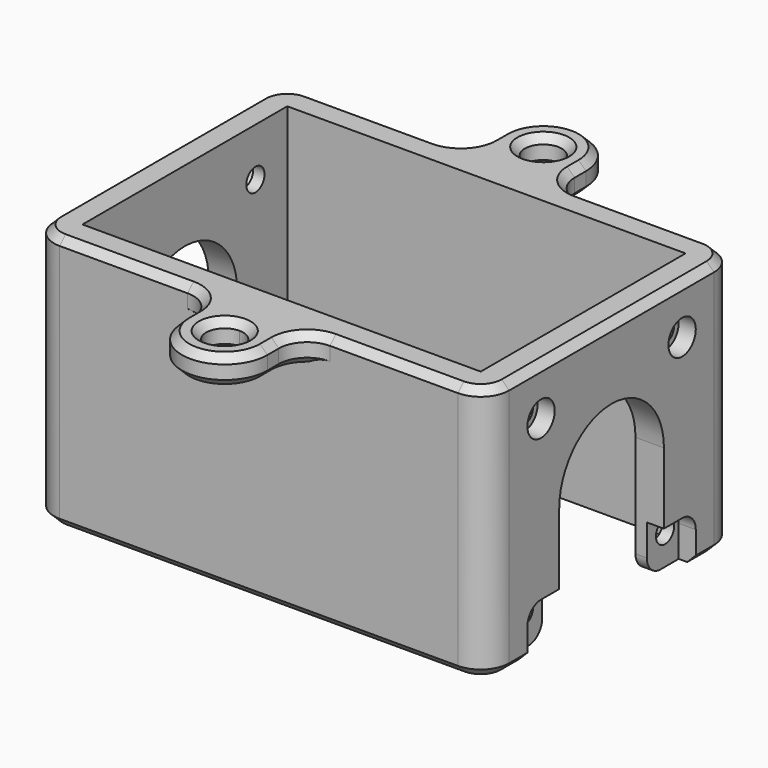
from build123d import *

# Parameters (mm, degrees)
F0_W          = 70
F0_H          = 45
F1_DEPTH      = 45
F2_R          = 2
F3_DEPTH      = 40.001
F3_DEPTH_BACK = 40.001
F5_R          = 3
F6_DEPTH      = 3
F7_R          = 3
F8_DEPTH      = 3
F9_R          = 3
F10_SIZE      = 1.5
F12_DEPTH     = 5
F13_R         = 5
F14_T1_DEPTH  = 22.5
F14_T3_DEPTH  = 22.5
F14_T5_DEPTH  = 2.5
F14_T7_DEPTH  = 45
F14_T9_DEPTH  = 2.5
F14_T16_ANGLE = 180
F14_T22_ANGLE = 128.3255006626
F14_T27_ANGLE = 90
F14_T29_ANGLE = 90
F14_T31_ANGLE = 180
F14_T33_ANGLE = 90
F14_T35_ANGLE = 90
F14_T37_ANGLE = 90
F14_T39_ANGLE = 90
F14_T41_ANGLE = 180
F14_T43_ANGLE = 90
F14_T45_ANGLE = 90
F14_T49_ANGLE = 128.3255006626
F14_T52_ANGLE = 180
F14_T56_ANGLE = 128.3255006626
F14_T61_ANGLE = 128.3255006626


# Not quite as in the source:
# - a fillet or chamfer that OpenCascade refuses, or shapes differently, is made with other operations: its cross-section is extruded or revolved along the edge and cut away or added


with BuildPart() as f1:
    # F0 (on Top) → F1 (new body)
    with BuildSketch(Plane.XY):
        with BuildLine():
            ThreePointArc((40, 22.5), (38.5355339059, 26.0355339059), (35, 27.5))
            Line((35, 27.5), (-35, 27.5))
            ThreePointArc((-35, 27.5), (-38.5355339059, 26.0355339059), (-40, 22.5))
            Line((-40, 22.5), (-40, -22.5))
            ThreePointArc((-40, -22.5), (-38.5355339059, -26.0355339059), (-35, -27.5))
            Line((-35, -27.5), (35, -27.5))
            ThreePointArc((35, -27.5), (38.5355339059, -26.0355339059), (40, -22.5))
            Line((40, -22.5), (40, 22.5))
        make_face()
        Rectangle(F0_W, F0_H, mode=Mode.SUBTRACT)
    extrude(amount=F1_DEPTH)

    # F2 (on Right) → F3 (cut, two sides)
    with BuildSketch(Plane.YZ) as f3_sk:
        with Locations((15.5, 36.5)):
            Circle(F2_R)
        with Locations((-15.5, 36.5)):
            Circle(F2_R)
        with Locations((15.5, 5.5)):
            Circle(F2_R)
        with Locations((-15.5, 5.5)):
            Circle(F2_R)
        with BuildLine():
            Line((11.5, 0), (11.5, 21))
            ThreePointArc((11.5, 21), (0, 32.5), (-11.5, 21))
            Line((-11.5, 21), (-11.5, 0))
            Line((-11.5, 0), (11.5, 0))
        make_face()
    extrude(amount=-F3_DEPTH, mode=Mode.SUBTRACT)
    extrude(f3_sk.sketch, amount=F3_DEPTH_BACK, mode=Mode.SUBTRACT)

    # F5 (on face) → F6 (cut)
    with BuildSketch(Plane.YZ.offset(40)):
        with Locations((-15.5, 36.5)):
            Circle(F5_R)
        with Locations((15.5, 36.5)):
            Circle(F5_R)
        with BuildLine():
            ThreePointArc((-15.5, 8.5), (-17.6213203436, 7.6213203436), (-18.5, 5.5))
            Line((-18.5, 5.5), (-18.5, 0))
            Line((-18.5, 0), (-11.5, 0))
            Line((-11.5, 0), (-11.5, 8.5))
            Line((-11.5, 8.5), (-15.5, 8.5))
        make_face()
        with BuildLine():
            Line((15.5, 8.5), (11.5, 8.5))
            Line((11.5, 8.5), (11.5, 0))
            Line((11.5, 0), (18.5, 0))
            Line((18.5, 0), (18.5, 5.5))
            ThreePointArc((18.5, 5.5), (17.6213203436, 7.6213203436), (15.5, 8.5))
        make_face()
    extrude(amount=-F6_DEPTH, mode=Mode.SUBTRACT)

    # F7 (on face) → F8 (cut)
    with BuildSketch(Plane(origin=(-40, 0, 0), x_dir=(0, -1, 0), z_dir=(-1, 0, 0))):
        with Locations((-15.5, 36.5)):
            Circle(F7_R)
        with Locations((15.5, 36.5)):
            Circle(F7_R)
        with BuildLine():
            Line((11.5, 0), (18.5, 0))
            Line((18.5, 0), (18.5, 5.5))
            ThreePointArc((18.5, 5.5), (17.6213203436, 7.6213203436), (15.5, 8.5))
            Line((15.5, 8.5), (11.5, 8.5))
            Line((11.5, 8.5), (11.5, 0))
        make_face()
        with BuildLine():
            Line((-11.5, 8.5), (-15.5, 8.5))
            ThreePointArc((-15.5, 8.5), (-17.6213203436, 7.6213203436), (-18.5, 5.5))
            Line((-18.5, 5.5), (-18.5, 0))
            Line((-18.5, 0), (-11.5, 0))
            Line((-11.5, 0), (-11.5, 8.5))
        make_face()
    extrude(amount=-F8_DEPTH, mode=Mode.SUBTRACT)

    # F9
    f9_edges = [f1.edges().sort_by_distance(p)[0] for p in [
        (36, 11.5, 0),
        (-36, 11.5, 0),
        (-36, -11.5, 0),
        (36, -11.5, 0),
    ]]
    fillet(f9_edges, radius=F9_R)

    # F10
    f10_edges = [f1.edges().sort_by_distance(p)[0] for p in [
        (-40, 20.5, 0),
        (-38.535534, -26.035534, 0),
        (-40, -20.5, 0),
        (0, -27.5, 0),
        (38.535534, -26.035534, 0),
        (40, -20.5, 0),
        (40, 20.5, 0),
        (38.535534, 26.035534, 0),
        (0, 27.5, 0),
        (-38.535534, 26.035534, 0),
    ]]
    chamfer(f10_edges, length=F10_SIZE)

    # F11 (on face) → F12 (join)
    with BuildSketch(Plane.XY.offset(45)):
        with BuildLine():
            Line((-7.5, 27.5), (0, 27.5))
            Line((0, 27.5), (7.5, 27.5))
            Line((7.5, 27.5), (7.5, 35))
            ThreePointArc((7.5, 35), (0, 42.5), (-7.5, 35))
            Line((-7.5, 35), (-7.5, 27.5))
        make_face()
        with BuildLine():
            ThreePointArc((0, 31.75), (-2.2980970389, 37.2980970389), (3.25, 35))
            ThreePointArc((3.25, 35), (2.2980970389, 32.7019029611), (0, 31.75))
        make_face(mode=Mode.SUBTRACT)
        with BuildLine():
            Line((7.5, -22.5), (0, -22.5))
            Line((0, -22.5), (-7.5, -22.5))
            Line((-7.5, -22.5), (-7.5, -35))
            ThreePointArc((-7.5, -35), (0, -42.5), (7.5, -35))
            Line((7.5, -35), (7.5, -22.5))
        make_face()
        with BuildLine():
            ThreePointArc((3.25, -35), (-2.2980970389, -37.2980970389), (0, -31.75))
            ThreePointArc((0, -31.75), (2.2980970389, -32.7019029611), (3.25, -35))
        make_face(mode=Mode.SUBTRACT)
    extrude(amount=-F12_DEPTH)

    # F13
    f13_edges = [f1.edges().sort_by_distance(p)[0] for p in [
        (7.5, 27.5, 42.5),
        (-7.5, 27.5, 42.5),
        (-7.5, -27.5, 42.5),
        (7.5, -27.5, 42.5),
    ]]
    fillet(f13_edges, radius=F13_R)

    # F14: chamfer of 1.3 on 34 edges, made by hand

    # F14_s2 → F14_t1 (cut)
    with BuildSketch(Plane.YZ.offset(12.5)):
        Polygon((-27.5, 43.7), (-26.2, 45), (-27.5, 45), align=None)
        Polygon((26.2, 45), (27.5, 43.7), (27.5, 45), align=None)
    extrude(amount=F14_T1_DEPTH, mode=Mode.SUBTRACT)

    # F14_s4 → F14_t3 (cut)
    with BuildSketch(Plane.YZ.offset(-35)):
        Polygon((-27.5, 43.7), (-26.2, 45), (-27.5, 45), align=None)
        Polygon((26.2, 45), (27.5, 43.7), (27.5, 45), align=None)
    extrude(amount=F14_T3_DEPTH, mode=Mode.SUBTRACT)

    # F14_s6 → F14_t5 (cut)
    with BuildSketch(Plane.XZ.offset(32.5)):
        Polygon((6.2, 45), (7.5, 43.7), (7.5, 45), align=None)
        Polygon((-6.2, 45), (-7.5, 43.7), (-7.5, 45), align=None)
        Polygon((-6.2, 40), (-7.5, 41.3), (-7.5, 40), align=None)
        Polygon((6.2, 40), (7.5, 41.3), (7.5, 40), align=None)
    extrude(amount=F14_T5_DEPTH, mode=Mode.SUBTRACT)

    # F14_s8 → F14_t7 (cut)
    with BuildSketch(Plane.XZ.offset(-22.5)):
        Polygon((38.7, 45), (40, 43.7), (40, 45), align=None)
        Polygon((-38.7, 45), (-40, 43.7), (-40, 45), align=None)
    extrude(amount=F14_T7_DEPTH, mode=Mode.SUBTRACT)

    # F14_s10 → F14_t9 (cut)
    with BuildSketch(Plane.XZ.offset(-35)):
        Polygon((6.2, 45), (7.5, 43.7), (7.5, 45), align=None)
        Polygon((-6.2, 45), (-7.5, 43.7), (-7.5, 45), align=None)
        Polygon((7.5, 41.3), (6.2, 40), (7.5, 40), align=None)
        Polygon((-7.5, 41.3), (-6.2, 40), (-7.5, 40), align=None)
    extrude(amount=F14_T9_DEPTH, mode=Mode.SUBTRACT)

    # F14_s11 → F14_t12 (revolve, cut)
    with BuildSketch(Plane.XZ.offset(35)):
        Polygon((4.55, 45), (3.25, 43.7), (3.25, 45), align=None)
    revolve(axis=Axis((0, -35, 45), (0, 0, -1)), mode=Mode.SUBTRACT)

    # F14_s13 → F14_t14 (revolve, cut)
    with BuildSketch(Plane.XZ.offset(-35)):
        Polygon((4.55, 45), (3.25, 43.7), (3.25, 45), align=None)
    revolve(axis=Axis((0, 35, 45), (0, 0, -1)), mode=Mode.SUBTRACT)

    # F14_s15 → F14_t16 (revolve, cut)
    with BuildSketch(Plane.XZ.offset(-35)):
        Polygon((7.5, 41.3), (6.2, 40), (7.5, 40), align=None)
    revolve(axis=Axis((0, 35, 40), (0, 0, 1)), revolution_arc=F14_T16_ANGLE, mode=Mode.SUBTRACT)

    # F14_s17 → F14_t18 (revolve, cut)
    with BuildSketch(Plane.XZ.offset(-35)):
        Polygon((3.25, 41.3), (4.55, 40), (3.25, 40), align=None)
    revolve(axis=Axis((0, 35, 40), (0, 0, -1)), mode=Mode.SUBTRACT)


with BuildPart() as f14_tool20:
    # F14_s21 → F14_t22 (revolve)
    with BuildSketch(Plane(origin=(-23.5039658434, -18.5793051911, 0), x_dir=(0, 0, 1), z_dir=(-0.7845004474, -0.6201282512, 0))):
        Polygon((40, -11.4446614013), (41.3, -12.7446614013), (40, -12.7446614013), align=None)
    revolve(axis=Axis((-12.5, -32.5, 40), (0, 0, -1)), revolution_arc=F14_T22_ANGLE)

    split(bisect_by=Plane.XZ.offset(27.5), keep=Keep.TOP)


with BuildPart() as f1_1:
    add(f1.part)

    # F14_t19: cut F14_tool20
    add(f14_tool20.part, mode=Mode.SUBTRACT)

    # F14_s24 → F14_t25 (revolve, cut)
    with BuildSketch(Plane.XZ.offset(35)):
        Polygon((4.55, 40), (3.25, 41.3), (3.25, 40), align=None)
    revolve(axis=Axis((0, -35, 40), (0, 0, -1)), mode=Mode.SUBTRACT)

    # F14_s26 → F14_t27 (revolve, cut)
    with BuildSketch(Plane.YZ.offset(12.5)):
        Polygon((-26.2, 45), (-27.5, 43.7), (-27.5, 45), align=None)
    revolve(axis=Axis((12.5, -32.5, 45), (0, 0, 1)), revolution_arc=F14_T27_ANGLE, mode=Mode.SUBTRACT)

    # F14_s28 → F14_t29 (revolve, cut)
    with BuildSketch(Plane.YZ.offset(35)):
        Polygon((-26.2, 45), (-27.5, 43.7), (-27.5, 45), align=None)
    revolve(axis=Axis((35, -22.5, 45), (0, 0, 1)), revolution_arc=F14_T29_ANGLE, mode=Mode.SUBTRACT)

    # F14_s30 → F14_t31 (revolve, cut)
    with BuildSketch(Plane.XZ.offset(35)):
        Polygon((-6.2, 45), (-7.5, 43.7), (-7.5, 45), align=None)
    revolve(axis=Axis((0, -35, 45), (0, 0, 1)), revolution_arc=F14_T31_ANGLE, mode=Mode.SUBTRACT)

    # F14_s32 → F14_t33 (revolve, cut)
    with BuildSketch(Plane.XZ.offset(-22.5)):
        Polygon((38.7, 45), (40, 43.7), (40, 45), align=None)
    revolve(axis=Axis((35, 22.5, 45), (0, 0, 1)), revolution_arc=F14_T33_ANGLE, mode=Mode.SUBTRACT)

    # F14_s34 → F14_t35 (revolve, cut)
    with BuildSketch(Plane.YZ.offset(-12.5)):
        Polygon((-26.2, 45), (-27.5, 43.7), (-27.5, 45), align=None)
    revolve(axis=Axis((-12.5, -32.5, 45), (0, 0, -1)), revolution_arc=F14_T35_ANGLE, mode=Mode.SUBTRACT)

    # F14_s36 → F14_t37 (revolve, cut)
    with BuildSketch(Plane.YZ.offset(12.5)):
        Polygon((26.2, 45), (27.5, 43.7), (27.5, 45), align=None)
    revolve(axis=Axis((12.5, 32.5, 45), (0, 0, -1)), revolution_arc=F14_T37_ANGLE, mode=Mode.SUBTRACT)

    # F14_s38 → F14_t39 (revolve, cut)
    with BuildSketch(Plane.XZ.offset(22.5)):
        Polygon((-38.7, 45), (-40, 43.7), (-40, 45), align=None)
    revolve(axis=Axis((-35, -22.5, 45), (0, 0, 1)), revolution_arc=F14_T39_ANGLE, mode=Mode.SUBTRACT)

    # F14_s40 → F14_t41 (revolve, cut)
    with BuildSketch(Plane.XZ.offset(-35)):
        Polygon((6.2, 45), (7.5, 43.7), (7.5, 45), align=None)
    revolve(axis=Axis((0, 35, 45), (0, 0, 1)), revolution_arc=F14_T41_ANGLE, mode=Mode.SUBTRACT)

    # F14_s42 → F14_t43 (revolve, cut)
    with BuildSketch(Plane.YZ.offset(-35)):
        Polygon((26.2, 45), (27.5, 43.7), (27.5, 45), align=None)
    revolve(axis=Axis((-35, 22.5, 45), (0, 0, 1)), revolution_arc=F14_T43_ANGLE, mode=Mode.SUBTRACT)

    # F14_s44 → F14_t45 (revolve, cut)
    with BuildSketch(Plane.YZ.offset(-12.5)):
        Polygon((26.2, 45), (27.5, 43.7), (27.5, 45), align=None)
    revolve(axis=Axis((-12.5, 32.5, 45), (0, 0, 1)), revolution_arc=F14_T45_ANGLE, mode=Mode.SUBTRACT)


with BuildPart() as f14_tool47:
    # F14_s48 → F14_t49 (revolve)
    with BuildSketch(Plane(origin=(23.5039658434, -18.5793051911, 0), x_dir=(0, 0, 1), z_dir=(0.7845004474, -0.6201282512, 0))):
        Polygon((41.3, 12.7446614013), (40, 11.4446614013), (40, 12.7446614013), align=None)
    revolve(axis=Axis((12.5, -32.5, 40), (0, 0, 1)), revolution_arc=F14_T49_ANGLE)

    split(bisect_by=Plane.XZ.offset(27.5), keep=Keep.TOP)


with BuildPart() as f1_2:
    add(f1_1.part)

    # F14_t46: cut F14_tool47
    add(f14_tool47.part, mode=Mode.SUBTRACT)

    # F14_s51 → F14_t52 (revolve, cut)
    with BuildSketch(Plane.XZ.offset(35)):
        Polygon((-6.2, 40), (-7.5, 41.3), (-7.5, 40), align=None)
    revolve(axis=Axis((0, -35, 40), (0, 0, 1)), revolution_arc=F14_T52_ANGLE, mode=Mode.SUBTRACT)


with BuildPart() as f14_tool54:
    # F14_s55 → F14_t56 (revolve)
    with BuildSketch(Plane(origin=(23.5039658434, 18.5793051911, 0), x_dir=(0, 0, 1), z_dir=(0.7845004474, 0.6201282512, 0))):
        Polygon((41.3, -12.7446614013), (40, -11.4446614013), (40, -12.7446614013), align=None)
    revolve(axis=Axis((12.5, 32.5, 40), (0, 0, -1)), revolution_arc=F14_T56_ANGLE)

    split(bisect_by=Plane.XZ.offset(-27.5), keep=Keep.BOTTOM)


with BuildPart() as f1_3:
    add(f1_2.part)

    # F14_t53: cut F14_tool54
    add(f14_tool54.part, mode=Mode.SUBTRACT)


with BuildPart() as f14_tool59:
    # F14_s60 → F14_t61 (revolve)
    with BuildSketch(Plane(origin=(-23.5039658434, 18.5793051911, 0), x_dir=(0, 0, 1), z_dir=(-0.7845004474, 0.6201282512, 0))):
        Polygon((41.3, 12.7446614013), (40, 11.4446614013), (40, 12.7446614013), align=None)
    revolve(axis=Axis((-12.5, 32.5, 40), (0, 0, 1)), revolution_arc=F14_T61_ANGLE)

    split(bisect_by=Plane.XZ.offset(-27.5), keep=Keep.BOTTOM)


with BuildPart() as f1_4:
    add(f1_3.part)

    # F14_t58: cut F14_tool59
    add(f14_tool59.part, mode=Mode.SUBTRACT)


solid = f1_4.part
